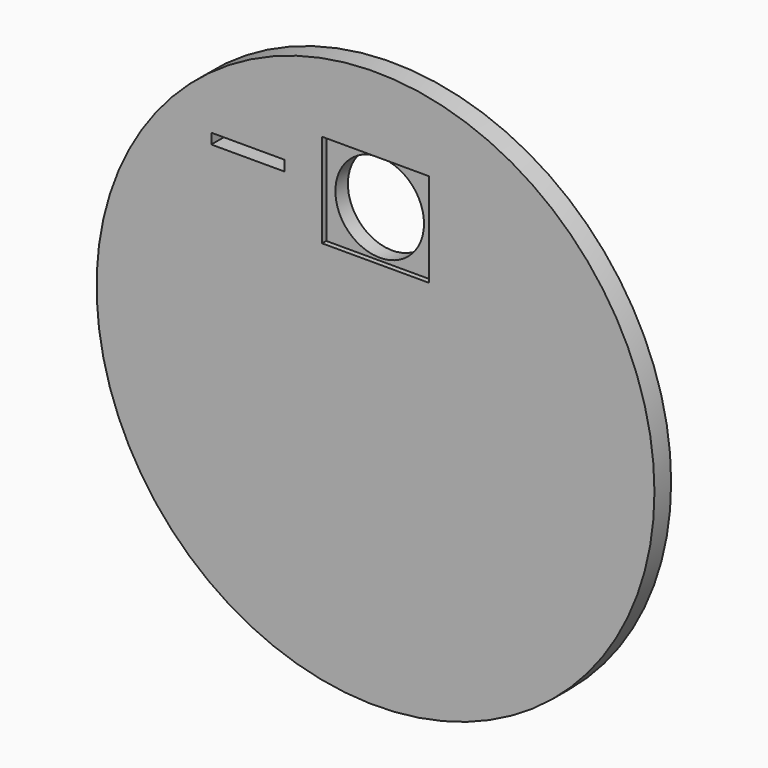
from build123d import *

# Parameters (mm, degrees)
F0_R     = 53.5
F0_R_2   = 8.5
F1_DEPTH = 4
F2_W     = 20.5
F2_H     = 18
F2_R     = 8.5
F3_DEPTH = 1
F4_W     = 14
F4_H     = 2
F5_DEPTH = 25


# Not quite as in the source:
# - a feature names something its author has since deleted; it is built from what else it names


with BuildPart() as f1:
    # F0 (on Front) → F1 (new body)
    with BuildSketch(Plane.XZ):
        Circle(F0_R)
        with Locations((0, 30.2263684571)):
            Circle(F0_R_2, mode=Mode.SUBTRACT)
    extrude(amount=F1_DEPTH)

    # F2 (on face) → F3 (cut)
    with BuildSketch(Plane.XZ.offset(4)):
        with Locations((0, 30.2263684571)):
            Rectangle(F2_W, F2_H)
        with Locations((0, 30.2263684571)):
            Circle(F2_R, mode=Mode.SUBTRACT)
    extrude(amount=-F3_DEPTH, mode=Mode.SUBTRACT)

    # F4 (on face) → F5 (cut)
    with BuildSketch(Plane.XZ.offset(4)):
        with Locations((-24.5, 32)):
            Rectangle(F4_W, F4_H)
    extrude(amount=-F5_DEPTH, mode=Mode.SUBTRACT)


solid = f1.part
